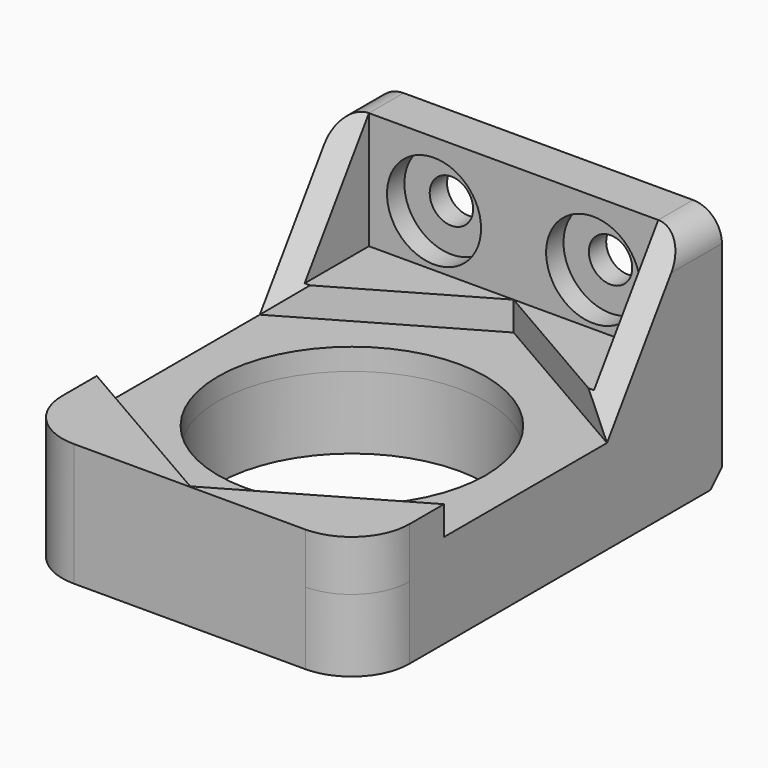
from build123d import *

# Parameters (mm, degrees)
F0_W           = 24
F0_H           = 11.6
F1_DEPTH       = 3
F3_D           = 3
F3_CBORE_D     = 6.5
F3_CBORE_DEPTH = 1.5
F4_DEPTH       = 28
F7_R           = 4
F8_R           = 9.25
F9_DEPTH       = 25
F10_DEPTH      = 5
F11_DEPTH      = 2
F2_W           = 2
F2_H           = 8.1
F12_REACH      = 36.3442607534
F5_W           = 2
F5_H           = 8.1
F13_REACH      = 36.3442607534
F14_SIZE       = 1
F15_R          = 2
F17_DEPTH      = 25


# Not quite as in the source:
# - a feature names something its author has since deleted; it is built from what else it names


with BuildPart() as f1:
    # F0 (on Front) → F1 (new body)
    with BuildSketch(Plane.XZ):
        with Locations((12, 5.8)):
            Rectangle(F0_W, F0_H)
    extrude(amount=F1_DEPTH)

    # F3 (through all)
    with Locations(Plane.XZ.offset(3)):
        with Locations((6.5, 7.1), (17.5, 7.1)):
            CounterBoreHole(F3_D / 2, F3_CBORE_D / 2, F3_CBORE_DEPTH)

    # F2 (on face) → F4 (join)
    with BuildSketch(Plane.XZ.offset(3)):
        Polygon((0, 3.5), (0, 0), (24, 0), (24, 3.5), (22, 3.5), (2, 3.5), align=None)
    extrude(amount=F4_DEPTH)

    # F7
    f7_edges = [f1.edges().sort_by_distance(p)[0] for p in [
        (24, -31, 1.75),
        (0, -31, 1.75),
    ]]
    fillet(f7_edges, radius=F7_R)

    # F8 (on face) → F9 (cut)
    with BuildSketch(Plane(origin=(0, 0, 0), x_dir=(1, 0, 0), z_dir=(0, 0, -1))):
        with Locations((12, 16.9718765144)):
            Circle(F8_R)
    extrude(amount=-F9_DEPTH, mode=Mode.SUBTRACT)

    # F10 (add): a face of the model
    f10_faces = [f1.faces().sort_by_distance(p)[0] for p in [
        (0.3920459157, -13.5, 0),
    ]]
    extrude(f10_faces, amount=F10_DEPTH)

    # F6 (on face) → F11 (cut)
    with BuildSketch(Plane.XY.offset(3.5)):
        Polygon((24, -24.0155497985), (24, -9.9282032303), (12, -3), (0, -9.9282032303), (0, -24.0155497985), (12, -30.9437530288), align=None)
    extrude(amount=-F11_DEPTH, mode=Mode.SUBTRACT)

    f12_end = Plane(origin=(6, -6.4641016151, 2.5), x_dir=(-0.8660254038, -0.5, 0), z_dir=(0.5, -0.8660254038, 0))
    # F2 (on face) → F12 (join, up to a plane its end follows)
    with BuildSketch(Plane.XZ.offset(3)):
        with Locations((1, 7.55)):
            Rectangle(F2_W, F2_H)
    f12_long = extrude(amount=F12_REACH, mode=Mode.PRIVATE)
    add(split(f12_long, bisect_by=f12_end, keep=Keep.BOTTOM, mode=Mode.PRIVATE))

    f13_end = Plane(origin=(18, -6.4641016151, 2.5), x_dir=(-0.8660254038, 0.5, 0), z_dir=(-0.5, -0.8660254038, 0))
    # F5 (on face) → F13 (join, up to a plane its end follows)
    with BuildSketch(Plane.XZ.offset(3)):
        with Locations((23, 7.55)):
            Rectangle(F5_W, F5_H)
    f13_long = extrude(amount=F13_REACH, mode=Mode.PRIVATE)
    add(split(f13_long, bisect_by=f13_end, keep=Keep.BOTTOM, mode=Mode.PRIVATE))

    # F14
    f14_edges = [f1.edges().sort_by_distance(p)[0] for p in [
        (12, 0, -5),
    ]]
    chamfer(f14_edges, length=F14_SIZE)

    # F15
    f15_edges = [f1.edges().sort_by_distance(p)[0] for p in [
        (24, -4.964102, 11.6),
        (0, -4.964102, 11.6),
    ]]
    fillet(f15_edges, radius=F15_R)

    # F16 (on face) → F17 (cut)
    with BuildSketch(Plane.YZ.offset(24)):
        Polygon((-9.9282032303, 11.6), (-9.9282032303, 1.5), (-3, 11.6), align=None)
    extrude(amount=-F17_DEPTH, mode=Mode.SUBTRACT)


solid = f1.part
